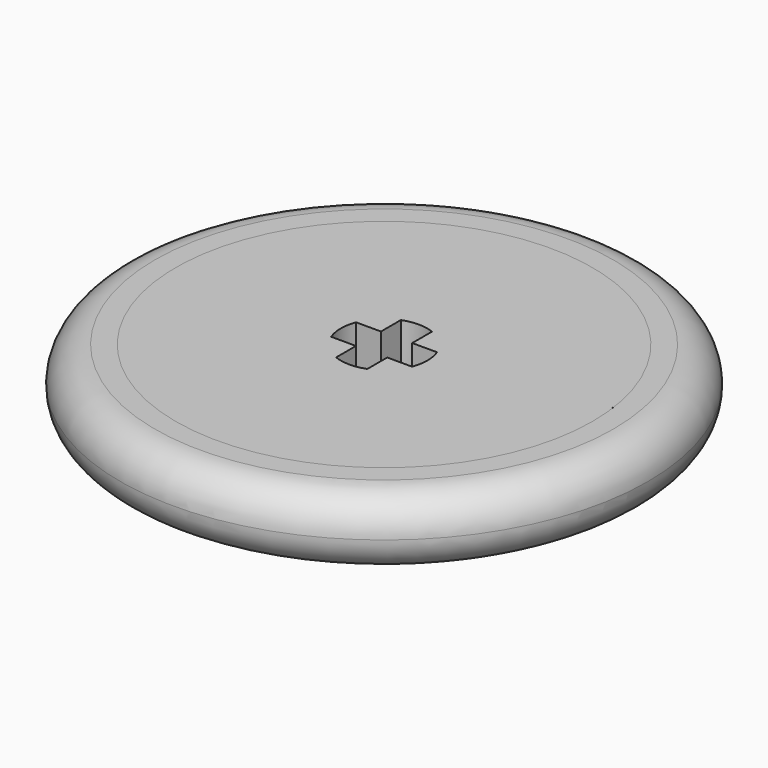
from build123d import *

# Parameters (mm, degrees)
F0_R     = 12
F1_DEPTH = 2
F0_R_2   = 15.2
F2_DEPTH = 2
F3_R     = 1.99999


# Not quite as in the source:
# - a fillet or chamfer is up to 0.001 mm smaller than in the source, because OpenCascade refuses the exact size


with BuildPart() as f1:
    # F0 (on Top) → F1 (new body, symmetric)
    with BuildSketch(Plane.XY):
        Circle(F0_R)
        with BuildLine():
            ThreePointArc((0.9, -2.3313088598), (0, -2.499), (-0.9, -2.3313088598))
            Line((-0.9, -2.3313088598), (-0.9, -0.9))
            Line((-0.9, -0.9), (-2.3313088598, -0.9))
            ThreePointArc((-2.3313088598, -0.9), (-2.499, 0), (-2.3313088598, 0.9))
            Line((-2.3313088598, 0.9), (-0.9, 0.9))
            Line((-0.9, 0.9), (-0.9, 2.3313088598))
            ThreePointArc((-0.9, 2.3313088598), (0, 2.499), (0.9, 2.3313088598))
            Line((0.9, 2.3313088598), (0.9, 0.9))
            Line((0.9, 0.9), (2.3313088598, 0.9))
            ThreePointArc((2.3313088598, 0.9), (2.499, 0), (2.3313088598, -0.9))
            Line((2.3313088598, -0.9), (0.9, -0.9))
            Line((0.9, -0.9), (0.9, -2.3313088598))
        make_face(mode=Mode.SUBTRACT)
    extrude(amount=F1_DEPTH, both=True)


with BuildPart() as f2:
    # F0 (on Top) → F2 (new body, symmetric)
    with BuildSketch(Plane.XY):
        Circle(F0_R_2)
        Circle(F0_R, mode=Mode.SUBTRACT)
    extrude(amount=F2_DEPTH, both=True)

    # F3 (radius 2 in the source; OpenCascade refuses exactly that, so slightly less here)
    f3_edges = [f2.edges().sort_by_distance(p)[0] for p in [
        (-15.2, 0, 2),
        (-15.2, 0, -2),
    ]]
    fillet(f3_edges, radius=F3_R)


solid = Compound([f1.part, f2.part])
